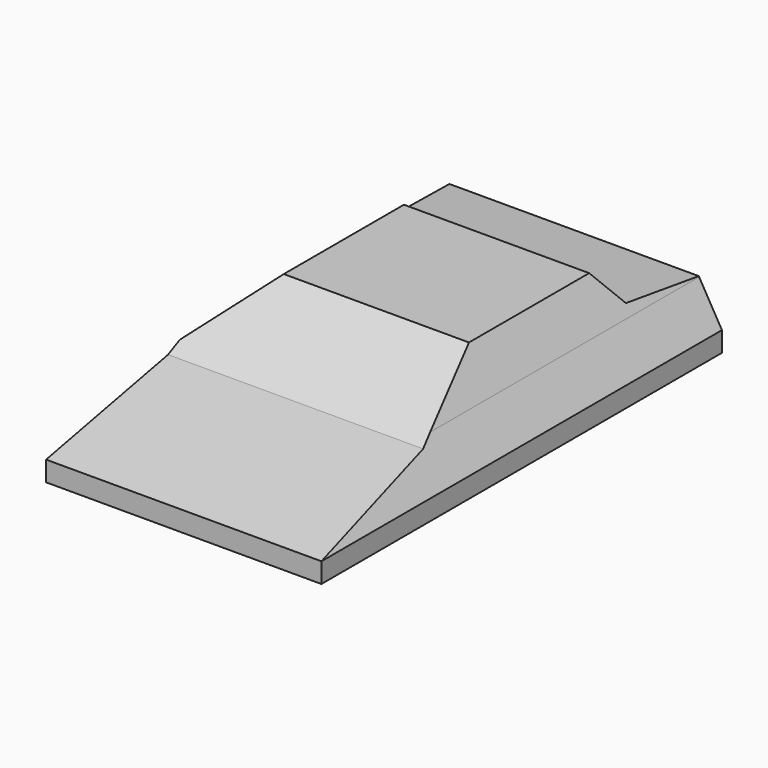
from build123d import *

# Parameters (mm, degrees)
F1_DEPTH      = 150
F1_DEPTH_BACK = 125
F3_DEPTH      = 2000


with BuildPart() as f1:
    # F0 (on Right) → F1 (new body, two sides)
    with BuildSketch(Plane.YZ) as f1_sk:
        Polygon((-150, 20), (-150, 0), (350, 0), (350, 60), (265.2117013931, 69.0981149673), (240.4940045903, 100), (90.4940045903, 100), (0, 51.8834842505), align=None)
    extrude(amount=F1_DEPTH)
    extrude(f1_sk.sketch, amount=-F1_DEPTH_BACK)

    # F2 (on face) → F3 (intersect)
    with BuildSketch(Plane(origin=(0, 350, 0), x_dir=(-1, 0, 0), z_dir=(0, 1, 0))):
        Polygon((122.7646524241, 59.4295346152), (80, 100), (-105, 100), (-127.2353475759, 59.4295346152), (-150, 20), (-150, 0), (125, 0), (125, 20), align=None)
    extrude(amount=-F3_DEPTH, mode=Mode.INTERSECT)


solid = f1.part
